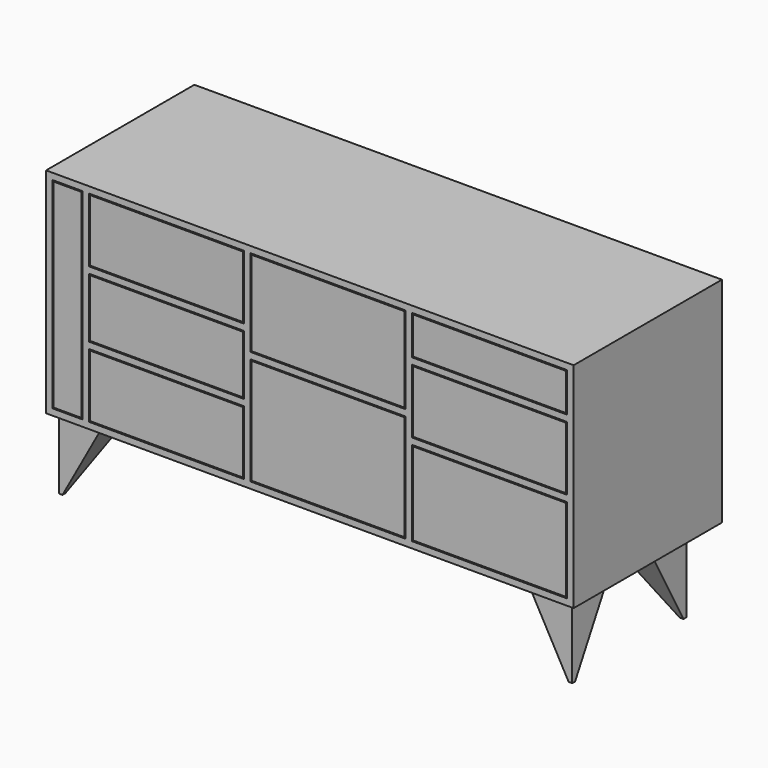
from build123d import *

# Parameters (mm, degrees)
F2_W        = 18
F2_H        = 564
F2_H_2      = 18
F2_W_2      = 84
F2_W_3      = 9
F2_W_4      = 435.3333333333
F3_DEPTH    = 520
F4_DEPTH    = 440
F5_W        = 78
F5_H        = 558
F6_DEPTH    = 12
F5_W_2      = 429.3333333333
F5_H_2      = 174
F5_H_3      = 162
F5_H_4      = 238
F5_H_5      = 296
F5_H_6      = 232
F5_H_7      = 104
F7_W        = 120
F7_H        = 120
F8_DEPTH    = 200
F9_SIZE2    = 109.99999
F9_SIZE     = 199.99999
F9_2_SIZE2  = 109.99999
F9_2_SIZE   = 199.99999
F10_SIZE2   = 199.99999
F10_SIZE    = 109.99999
F10_2_SIZE2 = 199.99999
F10_2_SIZE  = 109.99999
F11_SIZE2   = 109.99999
F11_SIZE    = 199.99999
F11_2_SIZE2 = 109.99999
F11_2_SIZE  = 199.99999
F12_SIZE2   = 109.99999
F12_SIZE    = 199.99999
F12_2_SIZE2 = 109.99999
F12_2_SIZE  = 199.99999


# Not quite as in the source:
# - a fillet or chamfer is up to 0.001 mm smaller than in the source, because OpenCascade refuses the exact size


with BuildPart() as f3:
    # F2 (on Front) → F3 (new body)
    with BuildSketch(Plane.XZ):
        with Locations((9, 300)):
            Rectangle(F2_W, F2_H)
        with Locations((9, 591)):
            Rectangle(F2_W, F2_H_2)
        with Locations((60, 591)):
            Rectangle(F2_W_2, F2_H_2)
        with Locations((115.5, 591)):
            Rectangle(F2_W_3, F2_H_2)
        with Locations((337.6666666667, 591)):
            Rectangle(F2_W_4, F2_H_2)
        with Locations((559.8333333333, 591)):
            Rectangle(F2_W_3, F2_H_2)
        with Locations((568.8333333333, 591)):
            Rectangle(F2_W_3, F2_H_2)
        with Locations((791, 591)):
            Rectangle(F2_W_4, F2_H_2)
        with Locations((1013.1666666667, 591)):
            Rectangle(F2_W_3, F2_H_2)
        with Locations((1022.1666666667, 591)):
            Rectangle(F2_W_3, F2_H_2)
        with Locations((1244.3333333333, 591)):
            Rectangle(F2_W_4, F2_H_2)
        with Locations((1475.5, 591)):
            Rectangle(F2_W_3, F2_H_2)
        with Locations((1475.5, 300)):
            Rectangle(F2_W_3, F2_H)
        with Locations((1475.5, 9)):
            Rectangle(F2_W_3, F2_H_2)
        with Locations((9, 9)):
            Rectangle(F2_W, F2_H_2)
        with Locations((106.5, 591)):
            Rectangle(F2_W_3, F2_H_2)
        with Locations((1466.5, 591)):
            Rectangle(F2_W_3, F2_H_2)
        Polygon((1462, 256), (1462, 18), (1471, 18), (1471, 582), (1462, 582), (1462, 472), (1462, 454), (1462, 274), align=None)
        with Locations((1466.5, 9)):
            Rectangle(F2_W_3, F2_H_2)
    extrude(amount=-F3_DEPTH)

    # F2 (on Front) → F4 (join)
    with BuildSketch(Plane.XZ):
        with Locations((1244.3333333333, 9)):
            Rectangle(F2_W_4, F2_H_2)
        with Locations((1022.1666666667, 9)):
            Rectangle(F2_W_3, F2_H_2)
        with Locations((1013.1666666667, 9)):
            Rectangle(F2_W_3, F2_H_2)
        with Locations((791, 9)):
            Rectangle(F2_W_4, F2_H_2)
        with Locations((568.8333333333, 9)):
            Rectangle(F2_W_3, F2_H_2)
        with Locations((559.8333333333, 9)):
            Rectangle(F2_W_3, F2_H_2)
        with Locations((337.6666666667, 9)):
            Rectangle(F2_W_4, F2_H_2)
        with Locations((115.5, 9)):
            Rectangle(F2_W_3, F2_H_2)
        with Locations((60, 9)):
            Rectangle(F2_W_2, F2_H_2)
        Polygon((111, 582), (111, 18), (120, 18), (120, 198), (120, 216), (120, 384), (120, 402), (120, 582), align=None)
        Polygon((555.3333333333, 198), (555.3333333333, 18), (564.3333333333, 18), (564.3333333333, 582), (555.3333333333, 582), (555.3333333333, 402), (555.3333333333, 384), (555.3333333333, 216), align=None)
        Polygon((564.3333333333, 582), (564.3333333333, 18), (573.3333333333, 18), (573.3333333333, 320), (573.3333333333, 338), (573.3333333333, 582), align=None)
        Polygon((1008.6666666667, 320), (1008.6666666667, 18), (1017.6666666667, 18), (1017.6666666667, 582), (1008.6666666667, 582), (1008.6666666667, 338), align=None)
        Polygon((1017.6666666667, 582), (1017.6666666667, 18), (1026.6666666667, 18), (1026.6666666667, 256), (1026.6666666667, 274), (1026.6666666667, 454), (1026.6666666667, 472), (1026.6666666667, 582), align=None)
        with Locations((106.5, 9)):
            Rectangle(F2_W_3, F2_H_2)
        with Locations((106.5, 300)):
            Rectangle(F2_W_3, F2_H)
        with Locations((337.6666666667, 393)):
            Rectangle(F2_W_4, F2_H_2)
        with Locations((337.6666666667, 207)):
            Rectangle(F2_W_4, F2_H_2)
        with Locations((791, 329)):
            Rectangle(F2_W_4, F2_H_2)
        with Locations((1244.3333333333, 463)):
            Rectangle(F2_W_4, F2_H_2)
        with Locations((1244.3333333333, 265)):
            Rectangle(F2_W_4, F2_H_2)
    extrude(amount=-F4_DEPTH)

    # F7 (on face) → F8 (join)
    with BuildSketch(Plane(origin=(0, 0, 0), x_dir=(1, 0, 0), z_dir=(0, 0, -1))):
        with Locations((80, -80)):
            Rectangle(F7_W, F7_H)
        with Locations((1400, -80)):
            Rectangle(F7_W, F7_H)
        with Locations((80, -360)):
            Rectangle(F7_W, F7_H)
        with Locations((1400, -360)):
            Rectangle(F7_W, F7_H)
    extrude(amount=F8_DEPTH)

    # F9 (size 200 and 110 in the source; OpenCascade refuses exactly that, so slightly less here)
    f9_edges = [f3.edges().sort_by_distance(p)[0] for p in [
        (140, 80, -200),
    ]]
    f9_side = f3.faces().sort_by_distance((140, 80, -100))[0]
    chamfer(f9_edges, length=F9_SIZE, length2=F9_SIZE2, reference=f9_side)

    # F9#2 (size 200 and 110 in the source; OpenCascade refuses exactly that, so slightly less here)
    f9_2_edges = [f3.edges().sort_by_distance(p)[0] for p in [
        (1340, 360, -200),
    ]]
    f9_2_side = f3.faces().sort_by_distance((1340, 360, -100))[0]
    chamfer(f9_2_edges, length=F9_2_SIZE, length2=F9_2_SIZE2, reference=f9_2_side)

    # F10 (size 110 and 200 in the source; OpenCascade refuses exactly that, so slightly less here)
    f10_edges = [f3.edges().sort_by_distance(p)[0] for p in [
        (25.000005, 140, -200),
    ]]
    f10_side = f3.faces().sort_by_distance((25.000005, 80, -200))[0]
    chamfer(f10_edges, length=F10_SIZE, length2=F10_SIZE2, reference=f10_side)

    # F10#2 (size 110 and 200 in the source; OpenCascade refuses exactly that, so slightly less here)
    f10_2_edges = [f3.edges().sort_by_distance(p)[0] for p in [
        (1454.999995, 300, -200),
    ]]
    f10_2_side = f3.faces().sort_by_distance((1454.999995, 360, -200))[0]
    chamfer(f10_2_edges, length=F10_2_SIZE, length2=F10_2_SIZE2, reference=f10_2_side)

    # F11 (size 200 and 110 in the source; OpenCascade refuses exactly that, so slightly less here)
    f11_edges = [f3.edges().sort_by_distance(p)[0] for p in [
        (140, 360, -200),
    ]]
    f11_side = f3.faces().sort_by_distance((140, 360, -100))[0]
    chamfer(f11_edges, length=F11_SIZE, length2=F11_SIZE2, reference=f11_side)

    # F11#2 (size 200 and 110 in the source; OpenCascade refuses exactly that, so slightly less here)
    f11_2_edges = [f3.edges().sort_by_distance(p)[0] for p in [
        (1340, 80, -200),
    ]]
    f11_2_side = f3.faces().sort_by_distance((1340, 80, -100))[0]
    chamfer(f11_2_edges, length=F11_2_SIZE, length2=F11_2_SIZE2, reference=f11_2_side)

    # F12 (size 200 and 110 in the source; OpenCascade refuses exactly that, so slightly less here)
    f12_edges = [f3.edges().sort_by_distance(p)[0] for p in [
        (25.000005, 300, -200),
    ]]
    f12_side = f3.faces().sort_by_distance((60.256413, 300, -71.794876))[0]
    chamfer(f12_edges, length=F12_SIZE, length2=F12_SIZE2, reference=f12_side)

    # F12#2 (size 200 and 110 in the source; OpenCascade refuses exactly that, so slightly less here)
    f12_2_edges = [f3.edges().sort_by_distance(p)[0] for p in [
        (1454.999995, 140, -200),
    ]]
    f12_2_side = f3.faces().sort_by_distance((1419.743587, 140, -71.794876))[0]
    chamfer(f12_2_edges, length=F12_2_SIZE, length2=F12_2_SIZE2, reference=f12_2_side)


with BuildPart() as f6:
    # F5 (on Front) → F6 (new body)
    with BuildSketch(Plane.XZ):
        with Locations((60, 300)):
            Rectangle(F5_W, F5_H)
    extrude(amount=-F6_DEPTH)


with BuildPart() as f6b:
    # F5 (on Front) → F6, piece 2 (new body)
    with BuildSketch(Plane.XZ):
        with Locations((337.6666666667, 492)):
            Rectangle(F5_W_2, F5_H_2)
    extrude(amount=-F6_DEPTH)


with BuildPart() as f6c:
    # F5 (on Front) → F6, piece 3 (new body)
    with BuildSketch(Plane.XZ):
        with Locations((337.6666666667, 300)):
            Rectangle(F5_W_2, F5_H_3)
    extrude(amount=-F6_DEPTH)


with BuildPart() as f6d:
    # F5 (on Front) → F6, piece 4 (new body)
    with BuildSketch(Plane.XZ):
        with Locations((337.6666666667, 108)):
            Rectangle(F5_W_2, F5_H_2)
    extrude(amount=-F6_DEPTH)


with BuildPart() as f6e:
    # F5 (on Front) → F6, piece 5 (new body)
    with BuildSketch(Plane.XZ):
        with Locations((791, 460)):
            Rectangle(F5_W_2, F5_H_4)
    extrude(amount=-F6_DEPTH)


with BuildPart() as f6f:
    # F5 (on Front) → F6, piece 6 (new body)
    with BuildSketch(Plane.XZ):
        with Locations((791, 169)):
            Rectangle(F5_W_2, F5_H_5)
    extrude(amount=-F6_DEPTH)


with BuildPart() as f6g:
    # F5 (on Front) → F6, piece 7 (new body)
    with BuildSketch(Plane.XZ):
        with Locations((1244.3333333333, 137)):
            Rectangle(F5_W_2, F5_H_6)
    extrude(amount=-F6_DEPTH)


with BuildPart() as f6h:
    # F5 (on Front) → F6, piece 8 (new body)
    with BuildSketch(Plane.XZ):
        with Locations((1244.3333333333, 364)):
            Rectangle(F5_W_2, F5_H_2)
    extrude(amount=-F6_DEPTH)


with BuildPart() as f6i:
    # F5 (on Front) → F6, piece 9 (new body)
    with BuildSketch(Plane.XZ):
        with Locations((1244.3333333333, 527)):
            Rectangle(F5_W_2, F5_H_7)
    extrude(amount=-F6_DEPTH)


solid = Compound([f3.part, f6.part, f6b.part, f6c.part, f6d.part, f6e.part, f6f.part, f6g.part, f6h.part, f6i.part])
